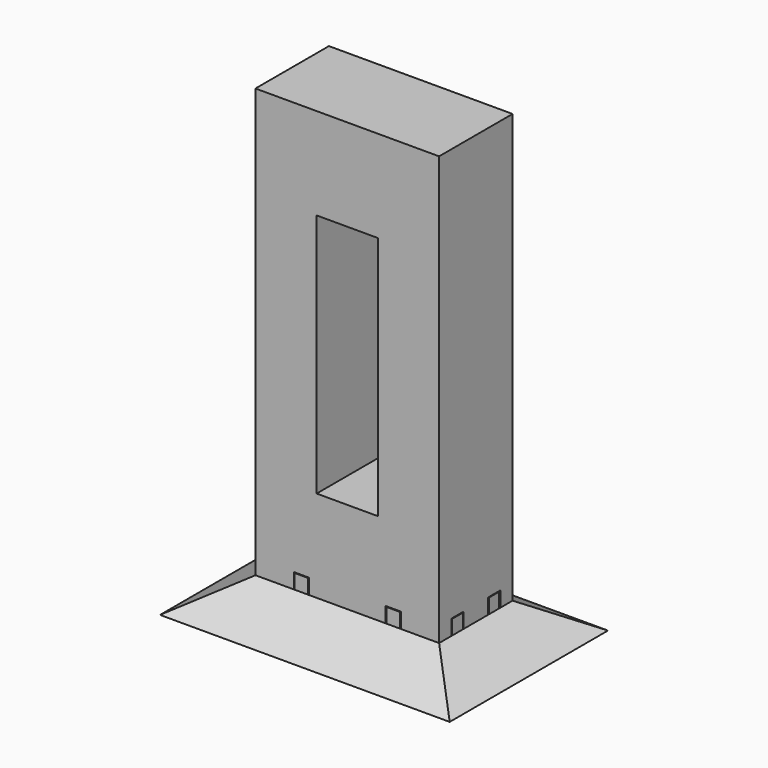
from build123d import *

# Parameters (mm, degrees)
F0_W     = 25.4
F0_H     = 101.6
F1_DEPTH = 38.1
F2_W     = 6.35
F2_H     = 6.35
F3_DEPTH = 76.201
F4_W     = 5.588
F4_H     = 6.731
F4_H_2   = 5.588
F4_W_2   = 16.3065173057
F4_H_3   = 13.462
F4_W_3   = 32.512
F4_W_4   = 16.2054826943
F4_H_4   = 5.334
F4_H_5   = 6.985
F5_DEPTH = 6.096
F6_W     = 76.2
F6_H     = 38.1
F7_DEPTH = 12.7
F7_TAPER = -60


with BuildPart() as f1:
    # F0 (on Front) → F1 (new body)
    with BuildSketch(Plane.XZ):
        Polygon((0, 177.8), (0, 0), (15.9255173057, 0), (15.9255173057, 6.35), (22.2755173057, 6.35), (22.2755173057, 0), (54.0255173057, 0), (54.0255173057, 6.35), (60.3755173057, 6.35), (60.3755173057, 0), (76.2, 0), (76.2, 177.8), align=None)
        with Locations((38.1, 88.9)):
            Rectangle(F0_W, F0_H, mode=Mode.SUBTRACT)
    extrude(amount=-F1_DEPTH)

    # F2 (on face) → F3 (cut, through all)
    with BuildSketch(Plane(origin=(0, 0, 0), x_dir=(0, -1, 0), z_dir=(-1, 0, 0))):
        with Locations((-28.575, 3.175)):
            Rectangle(F2_W, F2_H)
        with Locations((-9.525, 3.175)):
            Rectangle(F2_W, F2_H)
    extrude(amount=-F3_DEPTH, mode=Mode.SUBTRACT)


with BuildPart() as f5:
    # F4 (on Top) → F5 (new body)
    with BuildSketch(Plane.XY):
        with Locations((19.1005173057, 3.3655)):
            Rectangle(F4_W, F4_H)
        with Locations((19.1005173057, 9.525)):
            Rectangle(F4_W, F4_H_2)
        with Locations((8.1532586529, 9.525)):
            Rectangle(F4_W_2, F4_H_2)
        with Locations((19.1005173057, 19.05)):
            Rectangle(F4_W, F4_H_3)
        with Locations((38.1505173057, 9.525)):
            Rectangle(F4_W_3, F4_H_2)
        with Locations((57.2005173057, 9.525)):
            Rectangle(F4_W, F4_H_2)
        with Locations((57.2005173057, 3.3655)):
            Rectangle(F4_W, F4_H)
        with Locations((68.0972586529, 9.525)):
            Rectangle(F4_W_4, F4_H_2)
        with Locations((57.2005173057, 19.05)):
            Rectangle(F4_W, F4_H_3)
        with Locations((57.2005173057, 28.448)):
            Rectangle(F4_W, F4_H_4)
        with Locations((68.0972586529, 28.448)):
            Rectangle(F4_W_4, F4_H_4)
        with Locations((57.2005173057, 34.6075)):
            Rectangle(F4_W, F4_H_5)
        with Locations((38.1505173057, 28.448)):
            Rectangle(F4_W_3, F4_H_4)
        with Locations((19.1005173057, 28.448)):
            Rectangle(F4_W, F4_H_4)
        with Locations((19.1005173057, 34.6075)):
            Rectangle(F4_W, F4_H_5)
        with Locations((8.1532586529, 28.448)):
            Rectangle(F4_W_2, F4_H_4)
    extrude(amount=F5_DEPTH)

    # F6 (on face) → F7 (join)
    with BuildSketch(Plane(origin=(0, 0, 0), x_dir=(1, 0, 0), z_dir=(0, 0, -1))):
        with Locations((38.1, -19.05)):
            Rectangle(F6_W, F6_H)
    extrude(amount=F7_DEPTH, taper=F7_TAPER)


solid = Compound([f1.part, f5.part])
